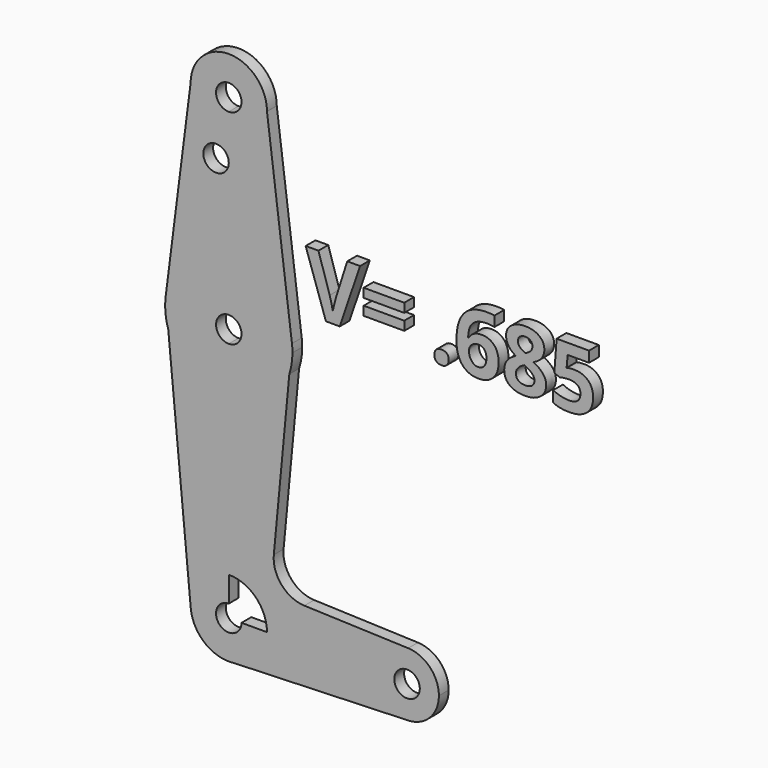
from build123d import *

# Parameters (mm, degrees)
F0_R         = 3.175
F0_TEXT_SIZE = 20.8765915078
F1_DEPTH     = 3.048


# Not quite as in the source:
# - Text() gives the source's letters only with a copy of the font that has no kerning and outlines rounded to 1/6400 em; it was checked with that copy


with BuildPart() as f1:
    # F0 (on Front) → F1 (new body)
    with BuildSketch(Plane.XZ):
        with BuildLine():
            ThreePointArc((-29.9494147476, 60.2143305507), (-29.9494021102, 60.2232886437), (-29.9493978977, 60.2322467446))
            ThreePointArc((-29.9493978977, 60.2322467446), (-39.4743978977, 69.7572467446), (-48.9993978977, 60.2322467446))
            ThreePointArc((-48.9993978977, 60.2322467446), (-46.2095899885, 53.4970546538), (-39.4743978977, 50.7072467446))
            ThreePointArc((-39.4743978977, 50.7072467446), (-32.7455431195, 53.4907232986), (-29.9494147476, 60.2143305507))
        make_face()
        with BuildLine():
            ThreePointArc((-36.2993978977, 60.2322467446), (-37.2293338675, 57.9871827144), (-39.4743978977, 57.0572467446))
            ThreePointArc((-39.4743978977, 57.0572467446), (-41.719461928, 62.4773107749), (-36.2993978977, 60.2322467446))
        make_face(mode=Mode.SUBTRACT)
        with BuildLine():
            ThreePointArc((-39.4743978977, 50.7072467446), (-46.2095899885, 53.4970546538), (-48.9993978977, 60.2322467446))
            Line((-48.9993978977, 60.2322467446), (-55.2225040142, 11.3092634646))
            ThreePointArc((-55.2225040142, 11.3092634646), (-49.9676087934, 21.2185920543), (-39.4743978977, 25.1810713261))
            Line((-39.4743978977, 25.1810713261), (-39.4743978977, 45.8312713261))
            Line((-39.4743978977, 45.8312713261), (-39.4743978977, 50.7072467446))
        make_face()
        with Locations((-42.6493978977, 45.8312713261)):
            Circle(F0_R, mode=Mode.SUBTRACT)
        with BuildLine():
            Line((-23.7263843398, 11.3099909802), (-29.9494147476, 60.2143305507))
            ThreePointArc((-29.9494147476, 60.2143305507), (-32.7455431195, 53.4907232986), (-39.4743978977, 50.7072467446))
            Line((-39.4743978977, 50.7072467446), (-39.4743978977, 45.8312713261))
            Line((-39.4743978977, 45.8312713261), (-39.4743978977, 25.1810713261))
            ThreePointArc((-39.4743978977, 25.1810713261), (-28.9814621671, 21.2188344294), (-23.7263843398, 11.3099909802))
        make_face()
        with BuildLine():
            Line((-54.5680983216, 4.3871453749), (-55.2225040142, 11.3092634646))
            ThreePointArc((-55.2225040142, 11.3092634646), (-55.2789284944, 7.8119369214), (-54.5680983216, 4.3871453749))
        make_face()
        with BuildLine():
            ThreePointArc((-39.4743978977, 25.1810713261), (-49.9676087934, 21.2185920543), (-55.2225040142, 11.3092634646))
            Line((-55.2225040142, 11.3092634646), (-54.5680983216, 4.3871453749))
            ThreePointArc((-54.5680983216, 4.3871453749), (-48.7998382499, -3.5411769099), (-39.4743978977, -6.5689286739))
            Line((-39.4743978977, -6.5689286739), (-39.4743978977, 6.1310713261))
            ThreePointArc((-39.4743978977, 6.1310713261), (-42.6493978977, 9.3060713261), (-39.4743978977, 12.4810713261))
            Line((-39.4743978977, 12.4810713261), (-39.4743978977, 25.1810713261))
        make_face()
        with BuildLine():
            Line((-24.3809009902, 4.3865209298), (-23.7263843398, 11.3099909802))
            ThreePointArc((-23.7263843398, 11.3099909802), (-28.9814621671, 21.2188344294), (-39.4743978977, 25.1810713261))
            Line((-39.4743978977, 25.1810713261), (-39.4743978977, 12.4810713261))
            ThreePointArc((-39.4743978977, 12.4810713261), (-37.2293338675, 11.5511353564), (-36.2993978977, 9.3060713261))
            ThreePointArc((-36.2993978977, 9.3060713261), (-37.2293338675, 7.0610072959), (-39.4743978977, 6.1310713261))
            Line((-39.4743978977, 6.1310713261), (-39.4743978977, -6.5689286739))
            ThreePointArc((-39.4743978977, -6.5689286739), (-30.1492233026, -3.5413698109), (-24.3809009902, 4.3865209298))
        make_face()
        with BuildLine():
            ThreePointArc((-23.5993978977, 9.3060713261), (-23.6311763151, 10.3100408895), (-23.7263843398, 11.3099909802))
            Line((-23.7263843398, 11.3099909802), (-24.3809009902, 4.3865209298))
            ThreePointArc((-24.3809009902, 4.3865209298), (-23.7959909568, 6.8154527692), (-23.5993978977, 9.3060713261))
        make_face()
        with BuildLine():
            ThreePointArc((-39.4743978977, -6.5689286739), (-48.7998382499, -3.5411769099), (-54.5680983216, 4.3871453749))
            Line((-54.5680983216, 4.3871453749), (-48.9571162557, -54.9642338982))
            ThreePointArc((-48.9571162557, -54.9642338982), (-46.5194175259, -47.6573458238), (-39.4743978977, -44.5427532554))
            Line((-39.4743978977, -44.5427532554), (-39.4743978977, -6.5689286739))
        make_face()
        with BuildLine():
            Line((-28.2481050899, -36.5207222211), (-24.3809009902, 4.3865209298))
            ThreePointArc((-24.3809009902, 4.3865209298), (-30.1492233026, -3.5413698109), (-39.4743978977, -6.5689286739))
            Line((-39.4743978977, -6.5689286739), (-39.4743978977, -44.5427532554))
            ThreePointArc((-39.4743978977, -44.5427532554), (-32.7392058069, -47.3325611646), (-29.9493978977, -54.0677532554))
            Line((-29.9493978977, -54.0677532554), (-2.9618978977, -54.0677532554))
            ThreePointArc((-2.9618978977, -54.0677532554), (-0.5363083824, -48.3561204714), (5.2580073768, -46.1352786408))
            Line((5.2580073768, -46.1352786408), (-20.6160514847, -45.2141322077))
            ThreePointArc((-20.6160514847, -45.2141322077), (-26.3076980008, -42.5140572732), (-28.2481050899, -36.5207222211))
        make_face()
        with BuildLine():
            ThreePointArc((-39.4743978977, -44.5427532554), (-46.5194175259, -47.6573458238), (-48.9571162557, -54.9642338982))
            ThreePointArc((-48.9571162557, -54.9642338982), (-46.0559781444, -60.9531309834), (-39.9423480029, -63.5812514395))
            Line((-39.9423480029, -63.5812514395), (-38.342876729, -63.5253049917))
            ThreePointArc((-38.342876729, -63.5253049917), (-32.3503764164, -60.3902482482), (-29.9493978977, -54.0677532554))
            Line((-29.9493978977, -54.0677532554), (-36.2993978977, -54.0677532554))
            ThreePointArc((-36.2993978977, -54.0677532554), (-41.719461928, -56.3128172856), (-39.4743978977, -50.8927532554))
            Line((-39.4743978977, -50.8927532554), (-39.4743978977, -44.5427532554))
        make_face()
        with BuildLine():
            Line((-38.342876729, -63.5253049917), (-39.9423480029, -63.5812514395))
            ThreePointArc((-39.9423480029, -63.5812514395), (-39.1414352267, -63.5869318365), (-38.342876729, -63.5253049917))
        make_face()
        with BuildLine():
            Line((-2.9618978977, -54.0677532554), (-29.9493978977, -54.0677532554))
            ThreePointArc((-29.9493978977, -54.0677532554), (-32.3503764164, -60.3902482482), (-38.342876729, -63.5253049917))
            Line((-38.342876729, -63.5253049917), (5.2530709948, -62.000402073))
            ThreePointArc((5.2530709948, -62.000402073), (-0.5380852717, -59.7776707497), (-2.9618978977, -54.0677532554))
        make_face()
        with BuildLine():
            ThreePointArc((12.9131021023, -54.0677532554), (10.6872348862, -48.5558427706), (5.2580073768, -46.1352786408))
            ThreePointArc((5.2580073768, -46.1352786408), (-0.5363083824, -48.3561204714), (-2.9618978977, -54.0677532554))
            ThreePointArc((-2.9618978977, -54.0677532554), (-0.5380852717, -59.7776707497), (5.2530709948, -62.000402073))
            ThreePointArc((5.2530709948, -62.000402073), (10.6855195966, -59.5814406293), (12.9131021023, -54.0677532554))
        make_face()
        with BuildLine():
            ThreePointArc((8.1506021023, -54.0677532554), (4.9756021023, -57.2427532554), (1.8006021023, -54.0677532554))
            ThreePointArc((1.8006021023, -54.0677532554), (4.9756021023, -50.8927532554), (8.1506021023, -54.0677532554))
        make_face(mode=Mode.SUBTRACT)
        with Locations((-20.3114729375, 18.9378280193)):
            Text('V= .685', F0_TEXT_SIZE, font='Open Sans', font_style=FontStyle.BOLD, text_align=(TextAlign.LEFT, TextAlign.BOTTOM))
    extrude(amount=F1_DEPTH)


solid = f1.part
